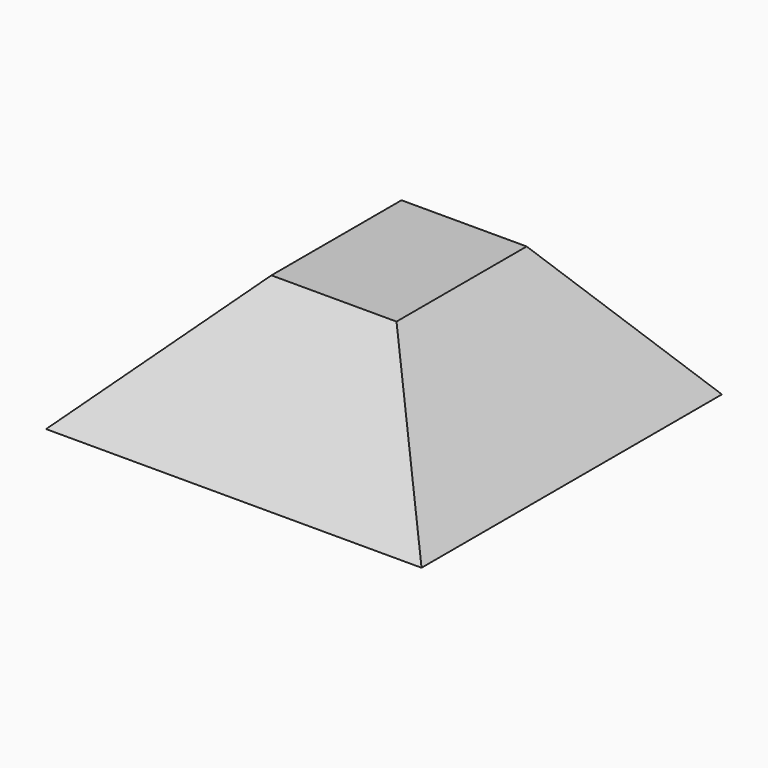
from build123d import *

# Parameters (mm, degrees)
F0_W     = 76.2
F0_H     = 76.2
F1_DEPTH = 25.4
F2_SIZE2 = 25.39999
F2_SIZE  = 25.39999
F3_SIZE2 = 17.785261
F3_SIZE  = 25.39999
F4_SIZE2 = 25.39999
F4_SIZE  = 25.39999
F5_SIZE2 = 25.39999
F5_SIZE  = 25.39999


# Not quite as in the source:
# - a fillet or chamfer is up to 0.001 mm smaller than in the source, because OpenCascade refuses the exact size


with BuildPart() as f1:
    # F0 (on Top) → F1 (new body)
    with BuildSketch(Plane.XY):
        with Locations((-5.1121336523, -3.4328531474)):
            Rectangle(F0_W, F0_H)
    extrude(amount=F1_DEPTH)

    # F2 (size 25.4 and 25.4 in the source; OpenCascade refuses exactly that, so slightly less here)
    f2_edges = [f1.edges().sort_by_distance(p)[0] for p in [
        (32.987866, -3.432853, 25.4),
    ]]
    chamfer(f2_edges, length=F2_SIZE, length2=F2_SIZE2)

    # F3 (size 25.4 and 17.7852714705 in the source; OpenCascade refuses exactly that, so slightly less here)
    f3_edges = [f1.edges().sort_by_distance(p)[0] for p in [
        (-17.812129, 34.667147, 25.4),
    ]]
    f3_side = f1.faces().sort_by_distance((-11.038795, 34.667147, 11.853333))[0]
    chamfer(f3_edges, length=F3_SIZE, length2=F3_SIZE2, reference=f3_side)

    # F4 (size 25.4 and 25.4 in the source; OpenCascade refuses exactly that, so slightly less here)
    f4_edges = [f1.edges().sort_by_distance(p)[0] for p in [
        (-43.212134, -12.325484, 25.4),
    ]]
    chamfer(f4_edges, length=F4_SIZE, length2=F4_SIZE2)

    # F5 (size 25.4 and 25.4 in the source; OpenCascade refuses exactly that, so slightly less here)
    f5_edges = [f1.edges().sort_by_distance(p)[0] for p in [
        (-5.112134, -41.532853, 25.4),
    ]]
    chamfer(f5_edges, length=F5_SIZE, length2=F5_SIZE2)


solid = f1.part
